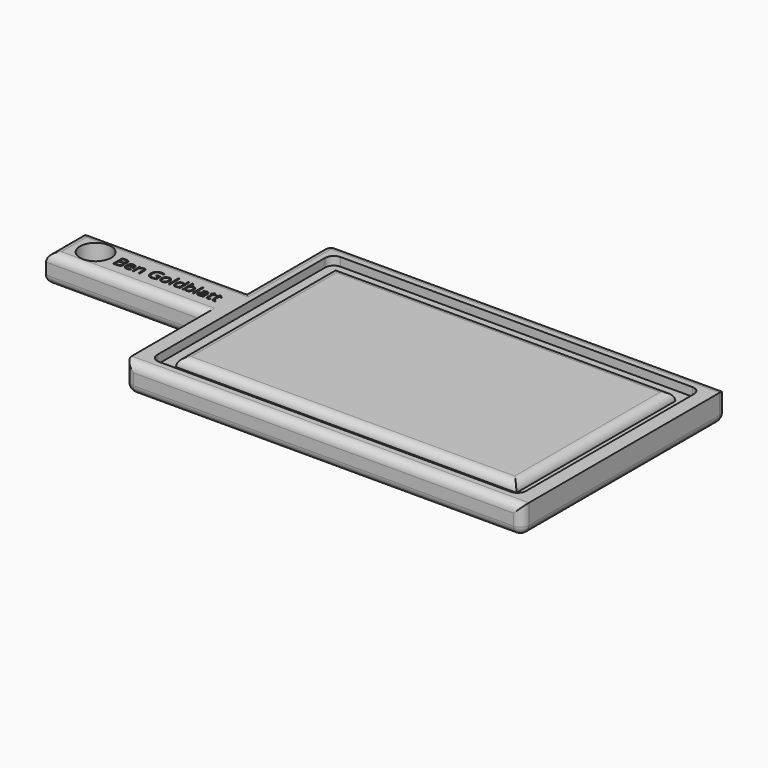
from build123d import *

# Parameters (mm, degrees)
F0_W          = 144.78
F0_H          = 43.18
F1_DEPTH      = 25.4
F2_R          = 13.97
F3_DEPTH      = 25.4
F6_DEPTH      = 7.62
F7_R          = 7.62
F8_R          = 7.62
F9_R          = 7.62
F10_R         = 7.62
F11_T1_DEPTH  = 304.7999950886
F11_T3_DEPTH  = 177.7999950886
F11_T5_DEPTH  = 36.83
F11_T7_DEPTH  = 340.36
F11_T9_DEPTH  = 393.7
F11_T11_DEPTH = 213.36
F11_T13_DEPTH = 85.09
F11_T15_DEPTH = 163.83
F11_T17_DEPTH = 85.09
F11_T19_DEPTH = 81.28
F11_S23_W     = 7.7724
F11_S23_H     = 7.7724
F11_T24_DEPTH = 7.7724
F11_S29_W     = 7.7724
F11_S29_H     = 7.7724
F11_T30_DEPTH = 7.7724
F11_S35_W     = 7.7724
F11_S35_H     = 7.7724
F11_T36_DEPTH = 7.7724
F11_S41_W     = 7.7724
F11_S41_H     = 7.7724
F11_T42_DEPTH = 7.7724
F11_T51_DEPTH = 104.14
F11_T55_DEPTH = 163.83
F11_T62_DEPTH = 104.14
F11_T66_DEPTH = 163.83
F12_T1_DEPTH  = 163.83
F12_T3_DEPTH  = 81.28
F12_T5_DEPTH  = 85.09
F12_S9_W      = 7.62
F12_S9_H      = 7.62
F12_T10_DEPTH = 7.62
F12_T17_DEPTH = 182.88
F12_T21_DEPTH = 104.14
F13_TEXT_SIZE = 14.565602751
F14_DEPTH     = 5.08


# Not quite as in the source:
# - a fillet or chamfer that OpenCascade refuses, or shapes differently, is made with other operations: its cross-section is extruded or revolved along the edge and cut away or added
# - Text() gives the source's letters only with a copy of the font that has no kerning and outlines rounded to 1/6400 em; it was checked with that copy


with BuildPart() as f1:
    # F0 (on Top) → F1 (new body)
    with BuildSketch(Plane.XY):
        Polygon((355.6, 228.6), (0, 228.6), (0, 135.89), (0, 92.71), (0, 0), (355.6, 0), align=None)
        with Locations((-72.39, 114.3)):
            Rectangle(F0_W, F0_H)
    extrude(amount=F1_DEPTH)

    # F2 (on face) → F3 (cut)
    with BuildSketch(Plane.XY.offset(25.4)):
        with Locations((-118.1148385341, 114.808)):
            Circle(F2_R)
    extrude(amount=-F3_DEPTH, mode=Mode.SUBTRACT)

    # F5 (on face) → F6 (cut)
    with BuildSketch(Plane.XY.offset(25.4)):
        Polygon((12.6999960899, 92.71), (12.6999960899, 12.6999960899), (342.9000039101, 12.6999960899), (342.9000039101, 215.9000039101), (12.6999960899, 215.9000039101), align=None)
        Polygon((25.4000024557, 25.4000024557), (25.4000024557, 92.71), (25.4000024557, 203.1999975443), (330.1999975443, 203.1999975443), (330.1999975443, 25.4000024557), align=None, mode=Mode.SUBTRACT)
    extrude(amount=-F6_DEPTH, mode=Mode.SUBTRACT)

    # F7
    f7_edges = [f1.edges().sort_by_distance(p)[0] for p in [
        (12.699996, 215.900004, 21.59),
    ]]
    fillet(f7_edges, radius=F7_R)

    # F8
    f8_edges = [f1.edges().sort_by_distance(p)[0] for p in [
        (342.900004, 215.900004, 21.59),
    ]]
    fillet(f8_edges, radius=F8_R)

    # F9
    f9_edges = [f1.edges().sort_by_distance(p)[0] for p in [
        (342.900004, 12.699996, 21.59),
    ]]
    fillet(f9_edges, radius=F9_R)

    # F10
    f10_edges = [f1.edges().sort_by_distance(p)[0] for p in [
        (12.699996, 12.699996, 21.59),
    ]]
    fillet(f10_edges, radius=F10_R)

    # F11: fillet of radius 7.62 on 19 edges, made by hand

    # F11_s2 → F11_t1 (cut)
    with BuildSketch(Plane.YZ.offset(25.4000024557)):
        with BuildLine():
            ThreePointArc((25.4000024557, 17.78), (27.6318487831, 23.1681536726), (33.0200024557, 25.4))
            Line((33.0200024557, 25.4), (25.4000024557, 25.4))
            Line((25.4000024557, 25.4), (25.4000024557, 17.78))
        make_face()
        with BuildLine():
            ThreePointArc((203.1999975443, 17.78), (200.9681512169, 23.1681536726), (195.5799975443, 25.4))
            Line((195.5799975443, 25.4), (203.1999975443, 25.4))
            Line((203.1999975443, 25.4), (203.1999975443, 17.78))
        make_face()
    extrude(amount=F11_T1_DEPTH, mode=Mode.SUBTRACT)

    # F11_s4 → F11_t3 (cut)
    with BuildSketch(Plane.XZ.offset(-203.1999975443)):
        with BuildLine():
            ThreePointArc((25.4000024557, 17.78), (27.6318487831, 23.1681536726), (33.0200024557, 25.4))
            Line((33.0200024557, 25.4), (25.4000024557, 25.4))
            Line((25.4000024557, 25.4), (25.4000024557, 17.78))
        make_face()
        with BuildLine():
            ThreePointArc((330.1999975443, 17.78), (327.9681512169, 23.1681536726), (322.5799975443, 25.4))
            Line((322.5799975443, 25.4), (330.1999975443, 25.4))
            Line((330.1999975443, 25.4), (330.1999975443, 17.78))
        make_face()
    extrude(amount=F11_T3_DEPTH, mode=Mode.SUBTRACT)

    # F11_s6 → F11_t5 (cut)
    with BuildSketch(Plane.XY.offset(7.62)):
        with BuildLine():
            ThreePointArc((7.62, 0), (2.2318463274, 2.2318463274), (0, 7.62))
            Line((0, 7.62), (0, 0))
            Line((0, 0), (7.62, 0))
        make_face()
        with BuildLine():
            ThreePointArc((355.6, 7.62), (353.3681536726, 2.2318463274), (347.98, 0))
            Line((347.98, 0), (355.6, 0))
            Line((355.6, 0), (355.6, 7.62))
        make_face()
        with BuildLine():
            ThreePointArc((347.98, 228.6), (353.3681536726, 226.3681536726), (355.6, 220.98))
            Line((355.6, 220.98), (355.6, 228.6))
            Line((355.6, 228.6), (347.98, 228.6))
        make_face()
        with BuildLine():
            ThreePointArc((7.62, 228.6), (2.2318463274, 226.3681536726), (0, 220.98))
            Line((0, 220.98), (0, 228.6))
            Line((0, 228.6), (7.62, 228.6))
        make_face()
    extrude(amount=F11_T5_DEPTH, mode=Mode.SUBTRACT)

    # F11_s8 → F11_t7 (cut)
    with BuildSketch(Plane.YZ.offset(7.62)):
        with BuildLine():
            ThreePointArc((0, 7.62), (2.2318463274, 2.2318463274), (7.62, 0))
            Line((7.62, 0), (0, 0))
            Line((0, 0), (0, 7.62))
        make_face()
        with BuildLine():
            ThreePointArc((228.6, 7.62), (226.3681536726, 2.2318463274), (220.98, 0))
            Line((220.98, 0), (228.6, 0))
            Line((228.6, 0), (228.6, 7.62))
        make_face()
    extrude(amount=F11_T7_DEPTH, mode=Mode.SUBTRACT)

    # F11_s10 → F11_t9 (cut)
    with BuildSketch(Plane.YZ.offset(-19.05)):
        with BuildLine():
            ThreePointArc((7.62, 25.4), (2.2318463274, 23.1681536726), (0, 17.78))
            Line((0, 17.78), (0, 25.4))
            Line((0, 25.4), (7.62, 25.4))
        make_face()
        with BuildLine():
            ThreePointArc((220.98, 25.4), (226.3681536726, 23.1681536726), (228.6, 17.78))
            Line((228.6, 17.78), (228.6, 25.4))
            Line((228.6, 25.4), (220.98, 25.4))
        make_face()
    extrude(amount=F11_T9_DEPTH, mode=Mode.SUBTRACT)

    # F11_s12 → F11_t11 (cut)
    with BuildSketch(Plane.XZ.offset(-220.98)):
        with BuildLine():
            ThreePointArc((355.6, 7.62), (353.3681536726, 2.2318463274), (347.98, 0))
            Line((347.98, 0), (355.6, 0))
            Line((355.6, 0), (355.6, 7.62))
        make_face()
    extrude(amount=F11_T11_DEPTH, mode=Mode.SUBTRACT)

    # F11_s14 → F11_t13 (cut)
    with BuildSketch(Plane.XZ.offset(-220.98)):
        with BuildLine():
            ThreePointArc((0, 7.62), (2.2318463274, 2.2318463274), (7.62, 0))
            Line((7.62, 0), (0, 0))
            Line((0, 0), (0, 7.62))
        make_face()
    extrude(amount=F11_T13_DEPTH, mode=Mode.SUBTRACT)

    # F11_s16 → F11_t15 (cut)
    with BuildSketch(Plane.YZ.offset(-163.83)):
        with BuildLine():
            ThreePointArc((135.89, 7.62), (133.6581536726, 2.2318463274), (128.27, 0))
            Line((128.27, 0), (135.89, 0))
            Line((135.89, 0), (135.89, 7.62))
        make_face()
        with BuildLine():
            ThreePointArc((92.71, 7.62), (94.9418463274, 2.2318463274), (100.33, 0))
            Line((100.33, 0), (92.71, 0))
            Line((92.71, 0), (92.71, 7.62))
        make_face()
    extrude(amount=F11_T15_DEPTH, mode=Mode.SUBTRACT)

    # F11_s18 → F11_t17 (cut)
    with BuildSketch(Plane.XZ.offset(-92.71)):
        with BuildLine():
            ThreePointArc((0, 7.62), (2.2318463274, 2.2318463274), (7.62, 0))
            Line((7.62, 0), (0, 0))
            Line((0, 0), (0, 7.62))
        make_face()
    extrude(amount=F11_T17_DEPTH, mode=Mode.SUBTRACT)

    # F11_s20 → F11_t19 (cut)
    with BuildSketch(Plane.XZ.offset(-154.94)):
        with BuildLine():
            ThreePointArc((-144.78, 7.62), (-142.5481536726, 2.2318463274), (-137.16, 0))
            Line((-137.16, 0), (-144.78, 0))
            Line((-144.78, 0), (-144.78, 7.62))
        make_face()
    extrude(amount=F11_T19_DEPTH, mode=Mode.SUBTRACT)


with BuildPart() as f11_tool22:
    # F11_s23 → F11_t24 (new body)
    with BuildSketch(Plane.XY.offset(7.62)):
        with Locations((3.7338, 3.7338)):
            Rectangle(F11_S23_W, F11_S23_H)
    extrude(amount=-F11_T24_DEPTH)

    # F11_s25 → F11_t26 (revolve, cut)
    with BuildSketch(Plane(origin=(7.62, 7.62, 7.62), x_dir=(0.7071067812, 0.7071067812, 0), z_dir=(-0.7071067812, 0.7071067812, 0))):
        with BuildLine():
            ThreePointArc((0, -7.62), (7.62, 0), (0, 7.62))
            Line((0, 7.62), (0, -7.62))
        make_face()
    revolve(axis=Axis((7.62, 7.62, 7.62), (0, 0, -1)), mode=Mode.SUBTRACT)


with BuildPart() as f1_1:
    add(f1.part)

    # F11_t21: cut F11_tool22
    add(f11_tool22.part, mode=Mode.SUBTRACT)


with BuildPart() as f11_tool28:
    # F11_s29 → F11_t30 (new body)
    with BuildSketch(Plane.YZ.offset(347.98)):
        with Locations((3.7338, 3.7338)):
            Rectangle(F11_S29_W, F11_S29_H)
    extrude(amount=F11_T30_DEPTH)

    # F11_s31 → F11_t32 (revolve, cut)
    with BuildSketch(Plane(origin=(347.98, 7.62, 7.62), x_dir=(0, 0.7071067812, 0.7071067812), z_dir=(0, 0.7071067812, -0.7071067812))):
        with BuildLine():
            ThreePointArc((0, -7.62), (7.62, 0), (0, 7.62))
            Line((0, 7.62), (0, -7.62))
        make_face()
    revolve(axis=Axis((347.98, 7.62, 7.62), (1, 0, 0)), mode=Mode.SUBTRACT)


with BuildPart() as f1_2:
    add(f1_1.part)

    # F11_t27: cut F11_tool28
    add(f11_tool28.part, mode=Mode.SUBTRACT)


with BuildPart() as f11_tool34:
    # F11_s35 → F11_t36 (new body)
    with BuildSketch(Plane.XZ.offset(-220.98)):
        with Locations((351.8662, 3.7338)):
            Rectangle(F11_S35_W, F11_S35_H)
    extrude(amount=-F11_T36_DEPTH)

    # F11_s37 → F11_t38 (revolve, cut)
    with BuildSketch(Plane(origin=(347.98, 220.98, 7.62), x_dir=(-0.7071067812, 0, 0.7071067812), z_dir=(-0.7071067812, 0, -0.7071067812))):
        with BuildLine():
            ThreePointArc((0, -7.62), (7.62, 0), (0, 7.62))
            Line((0, 7.62), (0, -7.62))
        make_face()
    revolve(axis=Axis((347.98, 220.98, 7.62), (0, 1, 0)), mode=Mode.SUBTRACT)


with BuildPart() as f1_3:
    add(f1_2.part)

    # F11_t33: cut F11_tool34
    add(f11_tool34.part, mode=Mode.SUBTRACT)


with BuildPart() as f11_tool40:
    # F11_s41 → F11_t42 (new body)
    with BuildSketch(Plane.YZ.offset(7.62)):
        with Locations((224.8662, 3.7338)):
            Rectangle(F11_S41_W, F11_S41_H)
    extrude(amount=-F11_T42_DEPTH)

    # F11_s43 → F11_t44 (revolve, cut)
    with BuildSketch(Plane(origin=(7.62, 220.98, 7.62), x_dir=(0, -0.7071067812, 0.7071067812), z_dir=(0, -0.7071067812, -0.7071067812))):
        with BuildLine():
            ThreePointArc((0, -7.62), (7.62, 0), (0, 7.62))
            Line((0, 7.62), (0, -7.62))
        make_face()
    revolve(axis=Axis((7.62, 220.98, 7.62), (-1, 0, 0)), mode=Mode.SUBTRACT)


with BuildPart() as f1_4:
    add(f1_3.part)

    # F11_t39: cut F11_tool40
    add(f11_tool40.part, mode=Mode.SUBTRACT)

    # F11_s45 → F11_t46 (revolve, cut)
    with BuildSketch(Plane.XZ.offset(-114.808)):
        with BuildLine():
            ThreePointArc((-104.1448385341, 7.62), (-101.9129922068, 2.2318463274), (-96.5248385341, 0))
            Line((-96.5248385341, 0), (-104.1448385341, 0))
            Line((-104.1448385341, 0), (-104.1448385341, 7.62))
        make_face()
    revolve(axis=Axis((-118.1148385341, 114.808, 0), (0, 0, 1)), mode=Mode.SUBTRACT)


with BuildPart() as f11_tool49:
    # F11_s50 → F11_t51 (new body)
    with BuildSketch(Plane.XZ.offset(-220.98)):
        with BuildLine():
            ThreePointArc((0, 7.62), (2.2318463274, 2.2318463274), (7.62, 0))
            Line((7.62, 0), (0, 0))
            Line((0, 0), (0, 7.62))
        make_face()
    extrude(amount=F11_T51_DEPTH)

    split(bisect_by=Plane.XZ.offset(-135.89), keep=Keep.TOP)


with BuildPart() as f11_tool53:
    # F11_s54 → F11_t55 (new body)
    with BuildSketch(Plane.YZ.offset(19.05)):
        with BuildLine():
            ThreePointArc((135.89, 7.62), (133.6581536726, 2.2318463274), (128.27, 0))
            Line((128.27, 0), (135.89, 0))
            Line((135.89, 0), (135.89, 7.62))
        make_face()
    extrude(amount=-F11_T55_DEPTH)

    split(bisect_by=Plane.YZ, keep=Keep.TOP)


with BuildPart() as f11_tool49_1:
    add(f11_tool49.part)

    # F11_t57: intersect F11_tool53
    add(f11_tool53.part, mode=Mode.INTERSECT)


with BuildPart() as f1_5:
    add(f1_4.part)

    # F11_t47: cut F11_tool49
    add(f11_tool49_1.part, mode=Mode.SUBTRACT)


with BuildPart() as f11_tool60:
    # F11_s61 → F11_t62 (new body)
    with BuildSketch(Plane.XZ.offset(-111.76)):
        with BuildLine():
            ThreePointArc((0, 7.62), (2.2318463274, 2.2318463274), (7.62, 0))
            Line((7.62, 0), (0, 0))
            Line((0, 0), (0, 7.62))
        make_face()
    extrude(amount=F11_T62_DEPTH)

    split(bisect_by=Plane.XZ.offset(-92.71), keep=Keep.BOTTOM)


with BuildPart() as f11_tool64:
    # F11_s65 → F11_t66 (new body)
    with BuildSketch(Plane.YZ.offset(-144.78)):
        with BuildLine():
            ThreePointArc((92.71, 7.62), (94.9418463274, 2.2318463274), (100.33, 0))
            Line((100.33, 0), (92.71, 0))
            Line((92.71, 0), (92.71, 7.62))
        make_face()
    extrude(amount=F11_T66_DEPTH)

    split(bisect_by=Plane.YZ, keep=Keep.TOP)


with BuildPart() as f11_tool60_1:
    add(f11_tool60.part)

    # F11_t68: intersect F11_tool64
    add(f11_tool64.part, mode=Mode.INTERSECT)


with BuildPart() as f1_6:
    add(f1_5.part)

    # F11_t58: cut F11_tool60
    add(f11_tool60_1.part, mode=Mode.SUBTRACT)

    # F12: fillet of radius 7.62 on 5 edges, made by hand

    # F12_s2 → F12_t1 (cut)
    with BuildSketch(Plane.YZ.offset(-163.83)):
        with BuildLine():
            ThreePointArc((100.33, 25.4), (94.9418463274, 23.1681536726), (92.71, 17.78))
            Line((92.71, 17.78), (92.71, 25.4))
            Line((92.71, 25.4), (100.33, 25.4))
        make_face()
        with BuildLine():
            ThreePointArc((128.27, 25.4), (133.6581536726, 23.1681536726), (135.89, 17.78))
            Line((135.89, 17.78), (135.89, 25.4))
            Line((135.89, 25.4), (128.27, 25.4))
        make_face()
    extrude(amount=F12_T1_DEPTH, mode=Mode.SUBTRACT)

    # F12_s4 → F12_t3 (cut)
    with BuildSketch(Plane.XZ.offset(-154.94)):
        with BuildLine():
            ThreePointArc((-137.16, 25.4), (-142.5481536726, 23.1681536726), (-144.78, 17.78))
            Line((-144.78, 17.78), (-144.78, 25.4))
            Line((-144.78, 25.4), (-137.16, 25.4))
        make_face()
    extrude(amount=F12_T3_DEPTH, mode=Mode.SUBTRACT)

    # F12_s6 → F12_t5 (cut)
    with BuildSketch(Plane.XZ.offset(-220.98)):
        with BuildLine():
            ThreePointArc((7.62, 25.4), (2.2318463274, 23.1681536726), (0, 17.78))
            Line((0, 17.78), (0, 25.4))
            Line((0, 25.4), (7.62, 25.4))
        make_face()
    extrude(amount=F12_T5_DEPTH, mode=Mode.SUBTRACT)


with BuildPart() as f12_tool8:
    # F12_s9 → F12_t10 (new body)
    with BuildSketch(Plane.XY.offset(17.78)):
        with Locations((3.81, 224.79)):
            Rectangle(F12_S9_W, F12_S9_H)
    extrude(amount=F12_T10_DEPTH)

    # F12_s11 → F12_t12 (revolve, cut)
    with BuildSketch(Plane(origin=(7.62, 220.98, 17.78), x_dir=(0.7071067812, -0.7071067812, 0), z_dir=(-0.7071067812, -0.7071067812, 0))):
        with BuildLine():
            ThreePointArc((0, -7.62), (7.62, 0), (0, 7.62))
            Line((0, 7.62), (0, -7.62))
        make_face()
    revolve(axis=Axis((7.62, 220.98, 17.78), (0, 0, 1)), mode=Mode.SUBTRACT)


with BuildPart() as f1_7:
    add(f1_6.part)

    # F12_t7: cut F12_tool8
    add(f12_tool8.part, mode=Mode.SUBTRACT)


with BuildPart() as f12_tool15:
    # F12_s16 → F12_t17 (new body)
    with BuildSketch(Plane.YZ.offset(19.05)):
        with BuildLine():
            ThreePointArc((128.27, 25.4), (133.6581536726, 23.1681536726), (135.89, 17.78))
            Line((135.89, 17.78), (135.89, 25.4))
            Line((135.89, 25.4), (128.27, 25.4))
        make_face()
    extrude(amount=-F12_T17_DEPTH)

    split(bisect_by=Plane.YZ, keep=Keep.TOP)


with BuildPart() as f12_tool19:
    # F12_s20 → F12_t21 (new body)
    with BuildSketch(Plane.XZ.offset(-220.98)):
        with BuildLine():
            ThreePointArc((7.62, 25.4), (2.2318463274, 23.1681536726), (0, 17.78))
            Line((0, 17.78), (0, 25.4))
            Line((0, 25.4), (7.62, 25.4))
        make_face()
    extrude(amount=F12_T21_DEPTH)

    split(bisect_by=Plane.XZ.offset(-135.89), keep=Keep.TOP)


with BuildPart() as f12_tool15_1:
    add(f12_tool15.part)

    # F12_t23: intersect F12_tool19
    add(f12_tool19.part, mode=Mode.INTERSECT)


with BuildPart() as f1_8:
    add(f1_7.part)

    # F12_t13: cut F12_tool15
    add(f12_tool15_1.part, mode=Mode.SUBTRACT)

    # F13 (on face) → F14 (cut)
    with BuildSketch(Plane.XY.offset(25.4)):
        with Locations((-99.06, 108.7329641532)):
            Text('Ben Goldblatt', F13_TEXT_SIZE, font='Open Sans', text_align=(TextAlign.LEFT, TextAlign.BOTTOM))
    extrude(amount=-F14_DEPTH, mode=Mode.SUBTRACT)


solid = f1_8.part
